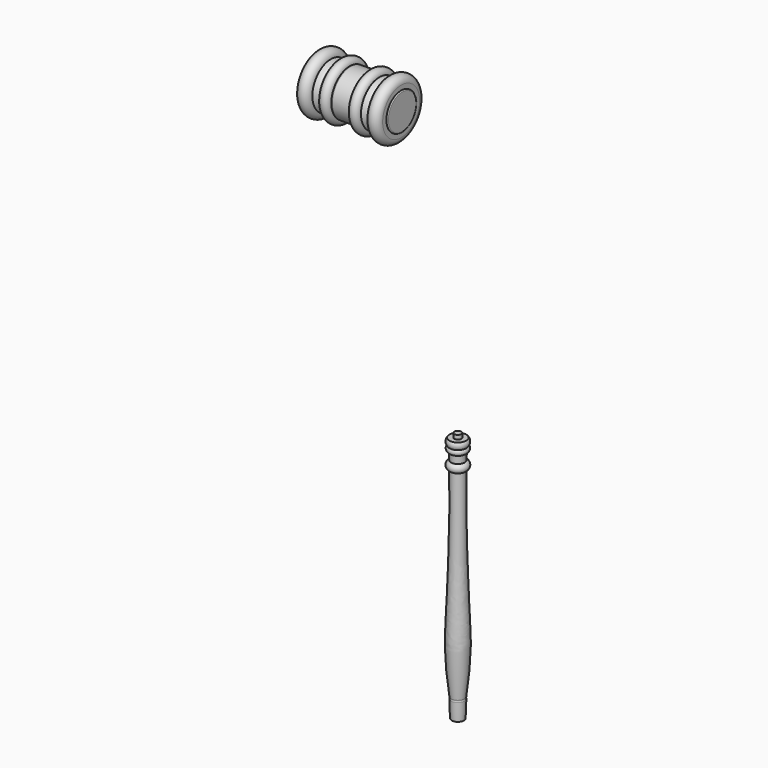
from build123d import *

# Parameters (mm, degrees)
F5_D     = 6.6548
F5_DEPTH = 21.972


# Not quite as in the source:
# - ends of sketch curves that miss each other by under 0.0002 mm in the source are joined


with BuildPart() as f1:
    # F0 (on Front) → F1 (revolve)
    with BuildSketch(Plane.XZ):
        with BuildLine():
            Line((-10.2444698859, 234.95), (-9.2283742104, 234.95))
            Line((-9.2283742104, 234.95), (-9.2283742104, 256.921))
            Line((-9.2283742104, 256.921), (-41.9944698859, 256.921))
            Line((-41.9944698859, 256.921), (-41.9944698859, 240.44275))
            ThreePointArc((-41.9944698859, 240.44275), (-41.6968903756, 239.7243295103), (-40.9784698859, 239.42675))
            Line((-40.9784698859, 239.42675), (-40.9784698859, 234.95))
            ThreePointArc((-40.9784698859, 234.95), (-34.6284698859, 228.6), (-28.2784698859, 234.95))
            add(Edge.make_bspline(
                [(-28.2784698859, 234.95), (-27.0824810676, 236.3563437226), (-24.6367592232, 239.2322281043), (-21.8357501873, 236.398168649), (-20.4044698859, 234.95)],
                knots=[0, 0, 0, 0, 0.4890126083, 1, 1, 1, 1], degree=3))
            ThreePointArc((-20.4044698859, 234.95), (-15.3244698859, 229.87), (-10.2444698859, 234.95))
        make_face()
    revolve(axis=Axis((-1.2273742104, 0, 256.921), (-1, 0, 0)))

    # F0 (on Front) → F2 (revolve)
    with BuildSketch(Plane.XZ):
        with BuildLine():
            Line((-10.2444698859, 234.95), (-9.2283742104, 234.95))
            Line((-9.2283742104, 234.95), (-9.2283742104, 256.921))
            Line((-9.2283742104, 256.921), (-41.9944698859, 256.921))
            Line((-41.9944698859, 256.921), (-41.9944698859, 240.44275))
            ThreePointArc((-41.9944698859, 240.44275), (-41.6968903756, 239.7243295103), (-40.9784698859, 239.42675))
            Line((-40.9784698859, 239.42675), (-40.9784698859, 234.95))
            ThreePointArc((-40.9784698859, 234.95), (-34.6284698859, 228.6), (-28.2784698859, 234.95))
            add(Edge.make_bspline(
                [(-28.2784698859, 234.95), (-27.0824810676, 236.3563437226), (-24.6367592232, 239.2322281043), (-21.8357501873, 236.398168649), (-20.4044698859, 234.95)],
                knots=[0, 0, 0, 0, 0.4890126083, 1, 1, 1, 1], degree=3))
            ThreePointArc((-20.4044698859, 234.95), (-15.3244698859, 229.87), (-10.2444698859, 234.95))
        make_face()
    revolve(axis=Axis((-1.2273742104, 0, 256.921), (-1, 0, 0)))


with BuildPart() as f1b:
    # F0 (on Front) → F1, piece 2 (revolve)
    with BuildSketch(Plane.XZ):
        with BuildLine():
            Line((6.7737214651, 256.921), (6.7737214651, 234.95))
            Line((6.7737214651, 234.95), (7.7897214651, 234.95))
            ThreePointArc((7.7897214651, 234.95), (12.8697214651, 229.87), (17.9497214651, 234.95))
            add(Edge.make_bspline(
                [(25.8237214651, 234.95), (24.6277326467, 236.3563437226), (22.1820108023, 239.2322281043), (19.3810017664, 236.398168649), (17.9497214651, 234.95)],
                knots=[0, 0, 0, 0, 0.4890126083, 1, 1, 1, 1], degree=3))
            ThreePointArc((25.8237214651, 234.95), (32.1737214651, 228.6), (38.5237214651, 234.95))
            Line((38.5237214651, 234.95), (38.5237214651, 239.42675))
            ThreePointArc((38.5237214651, 239.42675), (39.2421419547, 239.7243295103), (39.5397214651, 240.44275))
            Line((39.5397214651, 240.44275), (39.5397214651, 256.921))
            Line((39.5397214651, 256.921), (6.7737214651, 256.921))
        make_face()
    revolve(axis=Axis((-1.2273742104, 0, 256.921), (-1, 0, 0)))

    # F0 (on Front) → F2, piece 2 (revolve)
    with BuildSketch(Plane.XZ):
        with BuildLine():
            Line((6.7737214651, 256.921), (6.7737214651, 234.95))
            Line((6.7737214651, 234.95), (7.7897214651, 234.95))
            ThreePointArc((7.7897214651, 234.95), (12.8697214651, 229.87), (17.9497214651, 234.95))
            add(Edge.make_bspline(
                [(25.8237214651, 234.95), (24.6277326467, 236.3563437226), (22.1820108023, 239.2322281043), (19.3810017664, 236.398168649), (17.9497214651, 234.95)],
                knots=[0, 0, 0, 0, 0.4890126083, 1, 1, 1, 1], degree=3))
            ThreePointArc((25.8237214651, 234.95), (32.1737214651, 228.6), (38.5237214651, 234.95))
            Line((38.5237214651, 234.95), (38.5237214651, 239.42675))
            ThreePointArc((38.5237214651, 239.42675), (39.2421419547, 239.7243295103), (39.5397214651, 240.44275))
            Line((39.5397214651, 240.44275), (39.5397214651, 256.921))
            Line((39.5397214651, 256.921), (6.7737214651, 256.921))
        make_face()
    revolve(axis=Axis((-1.2273742104, 0, 256.921), (-1, 0, 0)))


with BuildPart() as f3:
    # F0 (on Front) → F3 (revolve)
    with BuildSketch(Plane.XZ):
        Polygon((-9.2283742104, 234.95), (-4.5298035257, 234.95), (-1.2273742104, 234.95), (6.7736257896, 234.95), (6.7737214651, 256.921), (-9.2283742104, 256.921), align=None)
    revolve(axis=Axis((-1.2273742104, 0, 256.921), (-1, 0, 0)))

    # F5 (through all, one way)
    with BuildSketch(Plane.XZ):
        with Locations((-1.2273742104, 256.921)):
            Circle(F5_D / 2)
    extrude(amount=-F5_DEPTH, mode=Mode.SUBTRACT)


with BuildPart() as f4:
    # F0 (on Front) → F4 (revolve)
    with BuildSketch(Plane.XZ):
        with BuildLine():
            ThreePointArc((86.1337266892, -215.0511991246), (86.3607392191, -216.0036991246), (86.1337266892, -216.9561991246))
            add(Edge.make_bspline(
                [(86.1337266892, -216.9561991246), (86.1299897573, -222.7984801777), (86.2199741445, -228.1975429416), (86.7052266892, -233.4661991246)],
                knots=[0, 0, 0, 0, 16.5198883849, 16.5198883849, 16.5198883849, 16.5198883849], degree=3))
            Line((86.7052266892, -233.4661991246), (92.4202266892, -233.4661991246))
            Line((92.4202266892, -233.4661991246), (92.4202266892, -25.1861991246))
            Line((92.4202266892, -25.1861991246), (92.4202266892, -17.3121991246))
            Line((92.4202266892, -17.3121991246), (92.4202266892, 1.4838008754))
            Line((92.4202266892, 1.4838008754), (92.4202266892, 5.4170577876))
            Line((92.4202266892, 5.4170577876), (89.1177973739, 5.4170577876))
            Line((89.1177973739, 5.4170577876), (89.1177973739, 1.4838008754))
            Line((89.1177973739, 1.4838008754), (84.4192266892, 1.4838008754))
            ThreePointArc((84.4192266892, 1.4838008754), (83.1852010196, -1.6911991246), (84.4192266892, -4.8661991246))
            ThreePointArc((84.4192266892, -4.8661991246), (83.3733644878, -7.4223986176), (84.6732266892, -9.8592699416))
            Line((84.6732266892, -9.8592699416), (85.6823071867, -9.8592699416))
            Line((85.6823071867, -9.8592699416), (85.9432266892, -17.3121991246))
            ThreePointArc((85.9432266892, -17.3121991246), (83.1492266892, -21.2491991246), (85.9432266892, -25.1861991246))
            add(Edge.make_bspline(
                [(86.1337266892, -215.0511991246), (84.8460040719, -205.7191707982), (81.8382387738, -176.5259328045), (84.1527333359, -138.910088313), (86.8161607127, -54.7569156535), (85.9432266892, -25.1861991246)],
                knots=[0, 0, 0, 0, 0.2576994007, 0.5405049731, 1, 1, 1, 1], degree=3))
        make_face()
    revolve(axis=Axis((92.4202266892, 0, -129.3261991246), (0, 0, 1)))


solid = Compound([f1.part, f1b.part, f3.part, f4.part])
